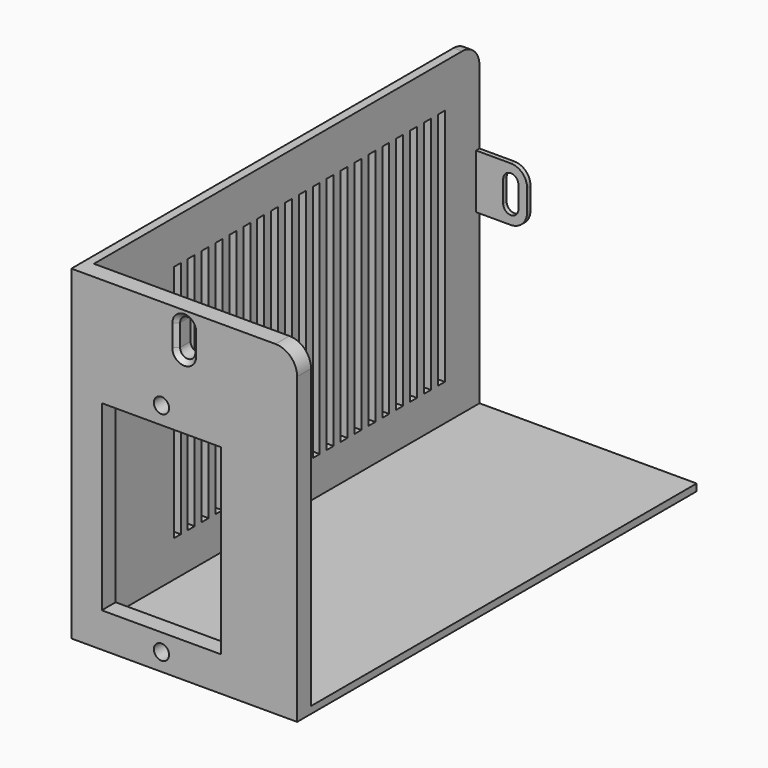
from build123d import *

# Parameters (mm, degrees)
F0_R     = 1.75
F0_W     = 27.5
F0_H     = 42
F1_DEPTH = 4
F3_W     = 110
F3_H     = 73.4
F3_W_2   = 2
F3_H_2   = 55
F3_W_3   = 1
F4_DEPTH = 2
F5_SIZE  = 1
F6_DEPTH = 50
F9_DEPTH = 1
F10_R    = 5


# Not quite as in the source:
# - a feature names something its author has since deleted; it is built from what else it names


with BuildPart() as f1:
    # F0 (on Front) → F1 (new body)
    with BuildSketch(Plane.XZ):
        Polygon((-22.9204972982, 50.6646189876), (-72.9204972982, 50.6646189876), (-74.9204972982, 50.6646189876), (-74.9204972982, -24.3353810124), (-72.9204972982, -24.3353810124), (-22.9204972982, -24.3353810124), align=None)
        with Locations((-54.1704972982, -20.3353810124)):
            Circle(F0_R, mode=Mode.SUBTRACT)
        with Locations((-54.1704972982, 4.6646189876)):
            Rectangle(F0_W, F0_H, mode=Mode.SUBTRACT)
        with Locations((-54.1704972982, 29.6646189876)):
            Circle(F0_R, mode=Mode.SUBTRACT)
        with BuildLine():
            Line((-50.6704972982, 42.1646189876), (-50.6704972982, 47.1646189876))
            ThreePointArc((-50.6704972982, 47.1646189876), (-48.9204972982, 48.9146189876), (-47.1704972982, 47.1646189876))
            Line((-47.1704972982, 47.1646189876), (-47.1704972982, 42.1646189876))
            ThreePointArc((-47.1704972982, 42.1646189876), (-48.9204972982, 40.4146189876), (-50.6704972982, 42.1646189876))
        make_face(mode=Mode.SUBTRACT)
    extrude(amount=F1_DEPTH)

    # F3 (on line) → F4 (join, through all)
    with BuildSketch(Plane(origin=(-72.9204972982, 0, 0), x_dir=(0, -1, 0), z_dir=(-1, 0, 0))):
        with Locations((-55, 13.9646189876)):
            Rectangle(F3_W, F3_H)
        with Locations((-100, 13.1646189876)):
            Rectangle(F3_W_2, F3_H_2, mode=Mode.SUBTRACT)
        with Locations((-96, 13.1646189876)):
            Rectangle(F3_W_2, F3_H_2, mode=Mode.SUBTRACT)
        with Locations((-92, 13.1646189876)):
            Rectangle(F3_W_2, F3_H_2, mode=Mode.SUBTRACT)
        with Locations((-88, 13.1646189876)):
            Rectangle(F3_W_2, F3_H_2, mode=Mode.SUBTRACT)
        with Locations((-84, 13.1646189876)):
            Rectangle(F3_W_2, F3_H_2, mode=Mode.SUBTRACT)
        with Locations((-80, 13.1646189876)):
            Rectangle(F3_W_2, F3_H_2, mode=Mode.SUBTRACT)
        with Locations((-76, 13.1646189876)):
            Rectangle(F3_W_2, F3_H_2, mode=Mode.SUBTRACT)
        with Locations((-72, 13.1646189876)):
            Rectangle(F3_W_2, F3_H_2, mode=Mode.SUBTRACT)
        with Locations((-68, 13.1646189876)):
            Rectangle(F3_W_2, F3_H_2, mode=Mode.SUBTRACT)
        with Locations((-64, 13.1646189876)):
            Rectangle(F3_W_2, F3_H_2, mode=Mode.SUBTRACT)
        with Locations((-60, 13.1646189876)):
            Rectangle(F3_W_2, F3_H_2, mode=Mode.SUBTRACT)
        with Locations((-56, 13.1646189876)):
            Rectangle(F3_W_2, F3_H_2, mode=Mode.SUBTRACT)
        with Locations((-52, 13.1646189876)):
            Rectangle(F3_W_2, F3_H_2, mode=Mode.SUBTRACT)
        with Locations((-48, 13.1646189876)):
            Rectangle(F3_W_2, F3_H_2, mode=Mode.SUBTRACT)
        with Locations((-44, 13.1646189876)):
            Rectangle(F3_W_2, F3_H_2, mode=Mode.SUBTRACT)
        with Locations((-40, 13.1646189876)):
            Rectangle(F3_W_2, F3_H_2, mode=Mode.SUBTRACT)
        with Locations((-36, 13.1646189876)):
            Rectangle(F3_W_2, F3_H_2, mode=Mode.SUBTRACT)
        with Locations((-32, 13.1646189876)):
            Rectangle(F3_W_2, F3_H_2, mode=Mode.SUBTRACT)
        with Locations((-28, 13.1646189876)):
            Rectangle(F3_W_2, F3_H_2, mode=Mode.SUBTRACT)
        with Locations((-24, 13.1646189876)):
            Rectangle(F3_W_2, F3_H_2, mode=Mode.SUBTRACT)
        with Locations((-110.5, 13.9646189876)):
            Rectangle(F3_W_3, F3_H)
        Polygon((0, -24.3353810124), (0, -22.7353810124), (-110, -22.7353810124), (-111, -22.7353810124), (-111, -24.3353810124), align=None)
    extrude(amount=F4_DEPTH)

    # F5
    f5_edges = [f1.edges().sort_by_distance(p)[0] for p in [
        (-47.170497, -4, 44.664619),
    ]]
    chamfer(f5_edges, length=F5_SIZE)

    # F3 (on line) → F6 (join, through all)
    with BuildSketch(Plane(origin=(-72.9204972982, 0, 0), x_dir=(0, -1, 0), z_dir=(-1, 0, 0))):
        Polygon((0, -24.3353810124), (0, -22.7353810124), (-110, -22.7353810124), (-111, -22.7353810124), (-111, -24.3353810124), align=None)
    extrude(amount=-F6_DEPTH)

    # F8 (on line) → F9 (join, through all)
    with BuildSketch(Plane(origin=(0, 111, 0), x_dir=(-1, 0, 0), z_dir=(0, 1, 0))):
        with BuildLine():
            Line((64.9204972982, 16.4146189876), (72.9204972982, 16.4146189876))
            Line((72.9204972982, 16.4146189876), (72.9204972982, 28.9146189876))
            Line((72.9204972982, 28.9146189876), (64.9204972982, 28.9146189876))
            ThreePointArc((64.9204972982, 28.9146189876), (62.2688468688, 27.816269417), (61.1704972982, 25.1646189876))
            Line((61.1704972982, 25.1646189876), (61.1704972982, 20.1646189876))
            ThreePointArc((61.1704972982, 20.1646189876), (62.2688468688, 17.5129685581), (64.9204972982, 16.4146189876))
        make_face()
        with BuildLine():
            Line((63.1704972982, 20.1646189876), (63.1704972982, 25.1646189876))
            ThreePointArc((63.1704972982, 25.1646189876), (64.9204972982, 26.9146189876), (66.6704972982, 25.1646189876))
            Line((66.6704972982, 25.1646189876), (66.6704972982, 20.1646189876))
            ThreePointArc((66.6704972982, 20.1646189876), (64.9204972982, 18.4146189876), (63.1704972982, 20.1646189876))
        make_face(mode=Mode.SUBTRACT)
    extrude(amount=-F9_DEPTH)

    # F10
    f10_edges = [f1.edges().sort_by_distance(p)[0] for p in [
        (-22.920497, -2, 50.664619),
        (-73.920497, 111, 50.664619),
    ]]
    fillet(f10_edges, radius=F10_R)


solid = f1.part
